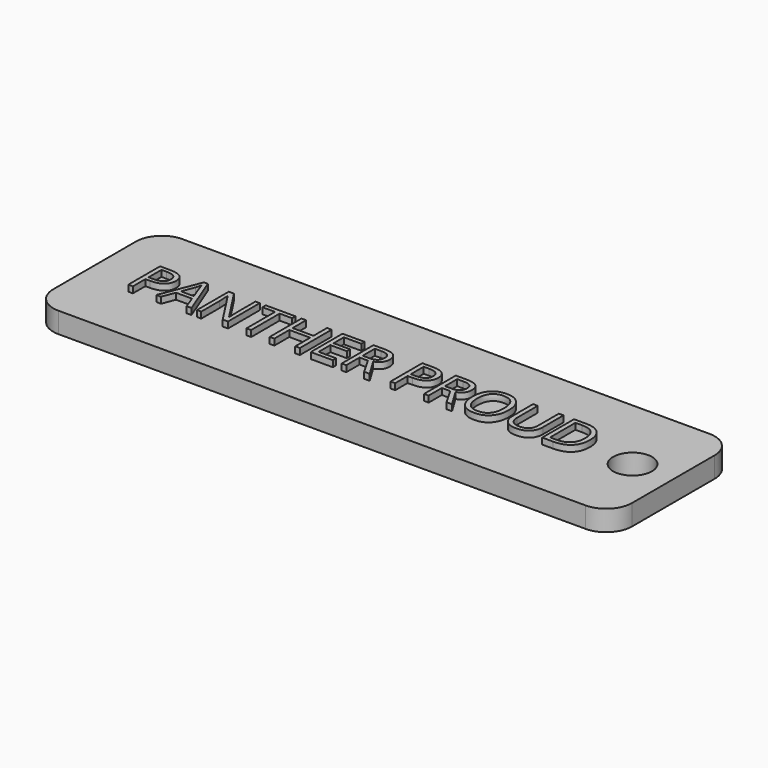
from build123d import *

# Parameters (mm, degrees)
F0_W         = 71.12
F0_H         = 19.05
F0_R         = 2.392877537
F1_DEPTH     = 2.54
F2_TEXT_SIZE = 6.8366500354
F3_DEPTH     = 0.762
F4_R         = 3.175


# Not quite as in the source:
# - Text() gives the source's letters only with a copy of the font that has no kerning and outlines rounded to 1/6400 em; it was checked with that copy


with BuildPart() as f1:
    # F0 (on Top) → F1 (new body)
    with BuildSketch(Plane.XY):
        Rectangle(F0_W, F0_H)
        with Locations((30.5415261537, 0)):
            Circle(F0_R, mode=Mode.SUBTRACT)
    extrude(amount=F1_DEPTH)

    # F2 (on face) → F3 (join)
    with BuildSketch(Plane.XY.offset(2.54)):
        with Locations((-30.2932420745, -2.2525054307)):
            Text('PANTHER PROUD', F2_TEXT_SIZE, font='Open Sans', text_align=(TextAlign.LEFT, TextAlign.BOTTOM))
    extrude(amount=F3_DEPTH)

    # F4
    f4_edges = [f1.edges().sort_by_distance(p)[0] for p in [
        (-35.56, -9.525, 1.27),
        (35.56, -9.525, 1.27),
        (35.56, 9.525, 1.27),
        (-35.56, 9.525, 1.27),
    ]]
    fillet(f4_edges, radius=F4_R)


solid = f1.part
